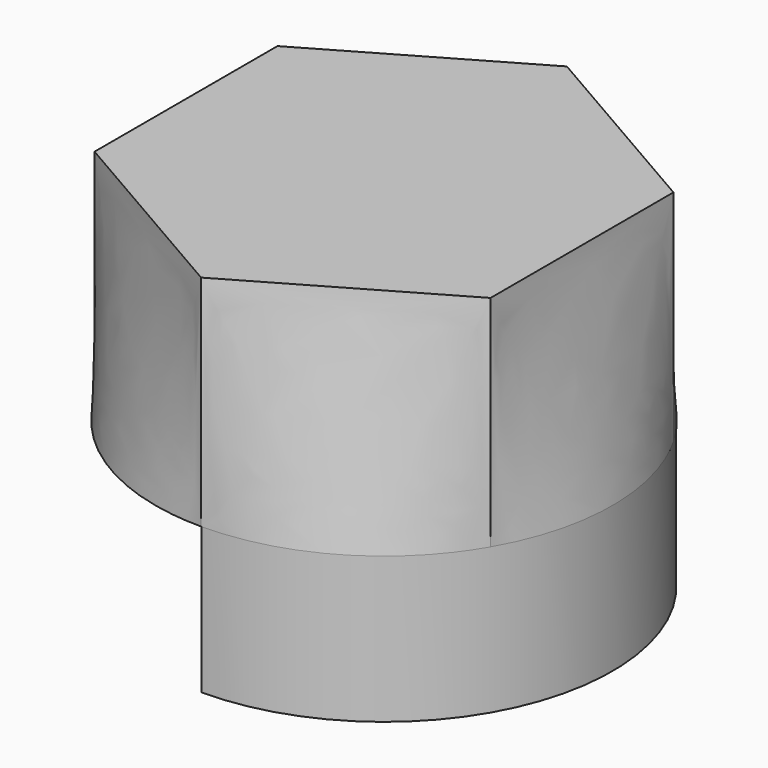
from build123d import *

# Parameters (mm, degrees)
F1_DEPTH = 20.32


# Not quite as in the source:
# - the arcs of a loft's sections are written as splines that run evenly, so that the points pair up as in the source's solid
# - a feature names something its author has since deleted; it is built from what else it names


with BuildPart() as f1:
    # F0 (on Top) → F1 (new body)
    with BuildSketch(Plane.XY):
        with BuildLine():
            ThreePointArc((0, -31.75), (31.75, 0), (0, 31.75))
            Line((0, 31.75), (0, -31.75))
        make_face()
    extrude(amount=F1_DEPTH)

    # F4 (on offset) → F6 section 0
    with BuildSketch(Plane.XY.offset(20.32)):
        with BuildLine():
            add(Edge.make_bspline(
                [(0, 31.7974612136), (-1.8499013065, 31.7974612136), (-3.6997740452, 31.63561832), (-7.3433683431, 30.9931543385), (-9.1370336348, 30.5125431721), (-12.6137108486, 29.2471361521), (-14.2966690809, 28.4623598401), (-17.5007921327, 26.6124585335), (-19.0219074714, 25.5473621069), (-21.8561207037, 23.169174829), (-23.169174829, 21.8561207037), (-25.5473621069, 19.0219074714), (-26.6124585335, 17.5007921327), (-27.5374091868, 15.8987306068)],
                knots=[0, 0, 0, 0, 0.1666666667, 0.1666666667, 0.3333333333, 0.3333333333, 0.5, 0.5, 0.6666666667, 0.6666666667, 0.8333333333, 0.8333333333, 1, 1, 1, 1], degree=3))
            add(Edge.make_bspline(
                [(-27.5374091868, 15.8987306068), (-28.4623598401, 14.2966690809), (-29.2471361521, 12.6137108486), (-30.5125431721, 9.1370336348), (-30.9931543385, 7.3433683431), (-31.63561832, 3.6997740452), (-31.7974612136, 1.8499013065), (-31.7974612136, -1.8499013065), (-31.63561832, -3.6997740452), (-30.9931543385, -7.3433683431), (-30.5125431721, -9.1370336348), (-29.2471361521, -12.6137108486), (-28.4623598401, -14.2966690809), (-27.5374091868, -15.8987306068)],
                knots=[0, 0, 0, 0, 0.1666666667, 0.1666666667, 0.3333333333, 0.3333333333, 0.5, 0.5, 0.6666666667, 0.6666666667, 0.8333333333, 0.8333333333, 1, 1, 1, 1], degree=3))
            add(Edge.make_bspline(
                [(-27.5374091868, -15.8987306068), (-26.6124585335, -17.5007921327), (-25.5473621069, -19.0219074714), (-23.169174829, -21.8561207037), (-21.8561207037, -23.169174829), (-19.0219074714, -25.5473621069), (-17.5007921327, -26.6124585335), (-14.2966690809, -28.4623598401), (-12.6137108486, -29.2471361521), (-9.1370336348, -30.5125431721), (-7.3433683431, -30.9931543385), (-3.6997740452, -31.63561832), (-1.8499013065, -31.7974612136), (0, -31.7974612136)],
                knots=[0, 0, 0, 0, 0.1666666667, 0.1666666667, 0.3333333333, 0.3333333333, 0.5, 0.5, 0.6666666667, 0.6666666667, 0.8333333333, 0.8333333333, 1, 1, 1, 1], degree=3))
            add(Edge.make_bspline(
                [(0, -31.7974612136), (1.8499013065, -31.7974612136), (3.6997740452, -31.63561832), (7.3433683431, -30.9931543385), (9.1370336348, -30.5125431721), (12.6137108486, -29.2471361521), (14.2966690809, -28.4623598401), (17.5007921327, -26.6124585335), (19.0219074714, -25.5473621069), (21.8561207037, -23.169174829), (23.169174829, -21.8561207037), (25.5473621069, -19.0219074714), (26.6124585335, -17.5007921327), (27.5374091868, -15.8987306068)],
                knots=[0, 0, 0, 0, 0.1666666667, 0.1666666667, 0.3333333333, 0.3333333333, 0.5, 0.5, 0.6666666667, 0.6666666667, 0.8333333333, 0.8333333333, 1, 1, 1, 1], degree=3))
            add(Edge.make_bspline(
                [(27.5374091868, -15.8987306068), (28.4623598401, -14.2966690809), (29.2471361521, -12.6137108486), (30.5125431721, -9.1370336348), (30.9931543385, -7.3433683431), (31.63561832, -3.6997740452), (31.7974612136, -1.8499013065), (31.7974612136, 1.8499013065), (31.63561832, 3.6997740452), (30.9931543385, 7.3433683431), (30.5125431721, 9.1370336348), (29.2471361521, 12.6137108486), (28.4623598401, 14.2966690809), (27.5374091868, 15.8987306068)],
                knots=[0, 0, 0, 0, 0.1666666667, 0.1666666667, 0.3333333333, 0.3333333333, 0.5, 0.5, 0.6666666667, 0.6666666667, 0.8333333333, 0.8333333333, 1, 1, 1, 1], degree=3))
            add(Edge.make_bspline(
                [(27.5374091868, 15.8987306068), (26.6124585335, 17.5007921327), (25.5473621069, 19.0219074714), (23.169174829, 21.8561207037), (21.8561207037, 23.169174829), (19.0219074714, 25.5473621069), (17.5007921327, 26.6124585335), (14.2966690809, 28.4623598401), (12.6137108486, 29.2471361521), (9.1370336348, 30.5125431721), (7.3433683431, 30.9931543385), (3.6997740452, 31.63561832), (1.8499013065, 31.7974612136), (0, 31.7974612136)],
                knots=[0, 0, 0, 0, 0.1666666667, 0.1666666667, 0.3333333333, 0.3333333333, 0.5, 0.5, 0.6666666667, 0.6666666667, 0.8333333333, 0.8333333333, 1, 1, 1, 1], degree=3))
        make_face()
    # F5 (on offset) → F6 section 1
    with BuildSketch(Plane.XY.offset(50.8)):
        Polygon((27.536238076, 15.8980544657), (0, 31.7961089313), (-27.536238076, 15.8980544657), (-27.536238076, -15.8980544657), (0, -31.7961089313), (27.536238076, -15.8980544657), align=None)
    loft(ruled=True)


solid = f1.part
